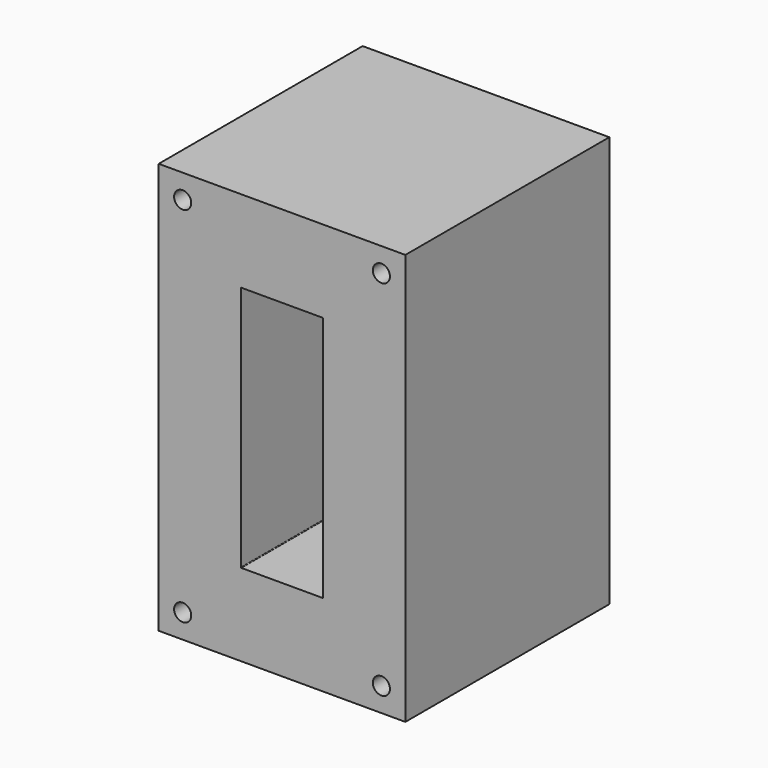
from build123d import *

# Parameters (mm, degrees)
F1_W     = 114.3
F1_H     = 190.5
F2_DEPTH = 118.11
F3_R     = 3.96875
F4_DEPTH = 118.11
F5_W     = 38.1
F5_H     = 114.3
F6_DEPTH = 118.11
F7_R     = 0.254


with BuildPart() as f2:
    # F1 (on Front) → F2 (new body)
    with BuildSketch(Plane.XZ):
        Rectangle(F1_W, F1_H)
    extrude(amount=-F2_DEPTH)

    # F3 (on face) → F4 (cut)
    with BuildSketch(Plane.XZ):
        with Locations((-46.0375, 84.1375)):
            Circle(F3_R)
        with Locations((46.0375, 84.1375)):
            Circle(F3_R)
        with Locations((-46.0375, -84.1375)):
            Circle(F3_R)
        with Locations((46.0375, -84.1375)):
            Circle(F3_R)
    extrude(amount=-F4_DEPTH, mode=Mode.SUBTRACT)

    # F5 (on face) → F6 (cut)
    with BuildSketch(Plane.XZ):
        Rectangle(F5_W, F5_H)
    extrude(amount=-F6_DEPTH, mode=Mode.SUBTRACT)

    # F7
    f7_edges = [f2.edges().sort_by_distance(p)[0] for p in [
        (-19.05, 59.055, 57.15),
        (19.05, 59.055, 57.15),
        (19.05, 59.055, -57.15),
        (-19.05, 59.055, -57.15),
    ]]
    fillet(f7_edges, radius=F7_R)


solid = f2.part
